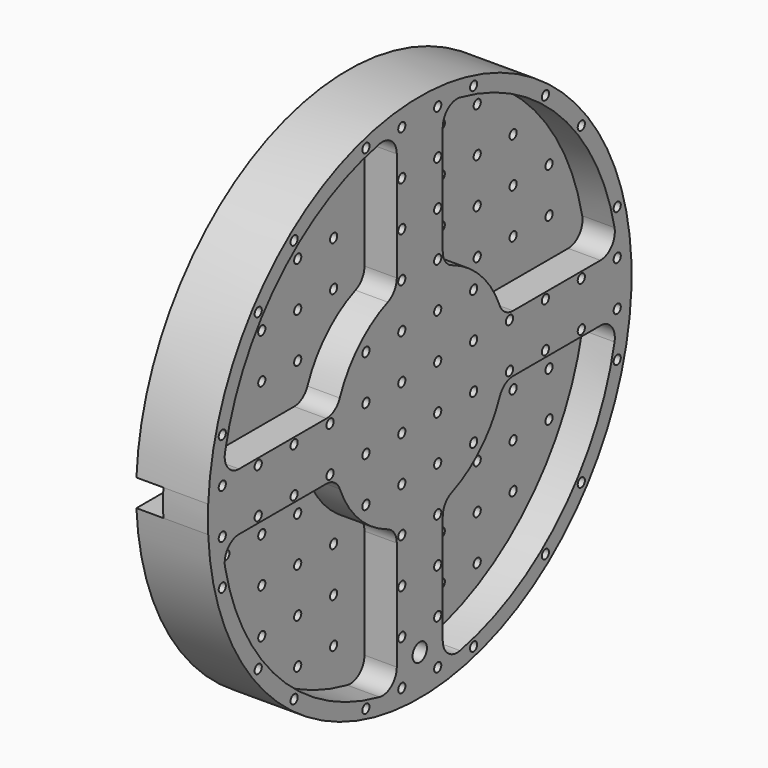
from build123d import *

# Parameters (mm, degrees)
F0_R     = 2.5
F0_R_2   = 5
F1_DEPTH = 40
F3_DEPTH = 15
F2_R     = 2.5
F4_DEPTH = 18


# Not quite as in the source:
# - a feature names something its author has since deleted; it is built from what else it names


with BuildPart() as f1:
    # F0 (on Right) → F1 (new body)
    with BuildSketch(Plane.YZ):
        with BuildLine():
            ThreePointArc((-147.3091986266, -7.5), (0, -147.5), (147.3091986266, -7.5))
            Line((147.3091986266, -7.5), (-147.3091986266, -7.5))
        make_face()
        with Locations((-87.5, -112.5)):
            Circle(F0_R, mode=Mode.SUBTRACT)
        with Locations((-112.5, -87.5)):
            Circle(F0_R, mode=Mode.SUBTRACT)
        with Locations((-87.5, -87.5)):
            Circle(F0_R, mode=Mode.SUBTRACT)
        with Locations((-37.5, -137.5)):
            Circle(F0_R, mode=Mode.SUBTRACT)
        with Locations((-62.5, -112.5)):
            Circle(F0_R, mode=Mode.SUBTRACT)
        with Locations((-37.5, -112.5)):
            Circle(F0_R, mode=Mode.SUBTRACT)
        with Locations((-12.5, -137.5)):
            Circle(F0_R, mode=Mode.SUBTRACT)
        with Locations((-12.5, -112.5)):
            Circle(F0_R, mode=Mode.SUBTRACT)
        with Locations((-62.5, -87.5)):
            Circle(F0_R, mode=Mode.SUBTRACT)
        with Locations((-37.5, -87.5)):
            Circle(F0_R, mode=Mode.SUBTRACT)
        with Locations((-12.5, -87.5)):
            Circle(F0_R, mode=Mode.SUBTRACT)
        with Locations((-112.5, -62.5)):
            Circle(F0_R, mode=Mode.SUBTRACT)
        with Locations((-137.5, -37.5)):
            Circle(F0_R, mode=Mode.SUBTRACT)
        with Locations((-112.5, -37.5)):
            Circle(F0_R, mode=Mode.SUBTRACT)
        with Locations((-87.5, -62.5)):
            Circle(F0_R, mode=Mode.SUBTRACT)
        with Locations((-87.5, -37.5)):
            Circle(F0_R, mode=Mode.SUBTRACT)
        with Locations((-137.5, -12.5)):
            Circle(F0_R, mode=Mode.SUBTRACT)
        with Locations((-112.5, -12.5)):
            Circle(F0_R, mode=Mode.SUBTRACT)
        with Locations((-87.5, -12.5)):
            Circle(F0_R, mode=Mode.SUBTRACT)
        with Locations((-62.5, -62.5)):
            Circle(F0_R, mode=Mode.SUBTRACT)
        with Locations((-37.5, -62.5)):
            Circle(F0_R, mode=Mode.SUBTRACT)
        with Locations((-62.5, -37.5)):
            Circle(F0_R, mode=Mode.SUBTRACT)
        with Locations((-37.5, -37.5)):
            Circle(F0_R, mode=Mode.SUBTRACT)
        with Locations((-12.5, -62.5)):
            Circle(F0_R, mode=Mode.SUBTRACT)
        with Locations((-12.5, -37.5)):
            Circle(F0_R, mode=Mode.SUBTRACT)
        with Locations((-62.5, -12.5)):
            Circle(F0_R, mode=Mode.SUBTRACT)
        with Locations((-37.5, -12.5)):
            Circle(F0_R, mode=Mode.SUBTRACT)
        with Locations((-12.5, -12.5)):
            Circle(F0_R, mode=Mode.SUBTRACT)
        with Locations((12.5, -137.5)):
            Circle(F0_R, mode=Mode.SUBTRACT)
        with Locations((0, -125)):
            Circle(F0_R_2, mode=Mode.SUBTRACT)
        with Locations((12.5, -112.5)):
            Circle(F0_R, mode=Mode.SUBTRACT)
        with Locations((37.5, -137.5)):
            Circle(F0_R, mode=Mode.SUBTRACT)
        with Locations((37.5, -112.5)):
            Circle(F0_R, mode=Mode.SUBTRACT)
        with Locations((62.5, -112.5)):
            Circle(F0_R, mode=Mode.SUBTRACT)
        with Locations((12.5, -87.5)):
            Circle(F0_R, mode=Mode.SUBTRACT)
        with Locations((37.5, -87.5)):
            Circle(F0_R, mode=Mode.SUBTRACT)
        with Locations((62.5, -87.5)):
            Circle(F0_R, mode=Mode.SUBTRACT)
        with Locations((87.5, -112.5)):
            Circle(F0_R, mode=Mode.SUBTRACT)
        with Locations((87.5, -87.5)):
            Circle(F0_R, mode=Mode.SUBTRACT)
        with Locations((112.5, -87.5)):
            Circle(F0_R, mode=Mode.SUBTRACT)
        with Locations((12.5, -62.5)):
            Circle(F0_R, mode=Mode.SUBTRACT)
        with Locations((12.5, -37.5)):
            Circle(F0_R, mode=Mode.SUBTRACT)
        with Locations((37.5, -62.5)):
            Circle(F0_R, mode=Mode.SUBTRACT)
        with Locations((62.5, -62.5)):
            Circle(F0_R, mode=Mode.SUBTRACT)
        with Locations((37.5, -37.5)):
            Circle(F0_R, mode=Mode.SUBTRACT)
        with Locations((62.5, -37.5)):
            Circle(F0_R, mode=Mode.SUBTRACT)
        with Locations((12.5, -12.5)):
            Circle(F0_R, mode=Mode.SUBTRACT)
        with Locations((37.5, -12.5)):
            Circle(F0_R, mode=Mode.SUBTRACT)
        with Locations((62.5, -12.5)):
            Circle(F0_R, mode=Mode.SUBTRACT)
        with Locations((87.5, -62.5)):
            Circle(F0_R, mode=Mode.SUBTRACT)
        with Locations((87.5, -37.5)):
            Circle(F0_R, mode=Mode.SUBTRACT)
        with Locations((112.5, -62.5)):
            Circle(F0_R, mode=Mode.SUBTRACT)
        with Locations((112.5, -37.5)):
            Circle(F0_R, mode=Mode.SUBTRACT)
        with Locations((137.5, -37.5)):
            Circle(F0_R, mode=Mode.SUBTRACT)
        with Locations((87.5, -12.5)):
            Circle(F0_R, mode=Mode.SUBTRACT)
        with Locations((112.5, -12.5)):
            Circle(F0_R, mode=Mode.SUBTRACT)
        with Locations((137.5, -12.5)):
            Circle(F0_R, mode=Mode.SUBTRACT)
        with BuildLine():
            Line((-147.3091986266, 7.5), (147.3091986266, 7.5))
            ThreePointArc((147.3091986266, 7.5), (0, 147.5), (-147.3091986266, 7.5))
        make_face()
        with Locations((-137.5, 12.5)):
            Circle(F0_R, mode=Mode.SUBTRACT)
        with Locations((-112.5, 12.5)):
            Circle(F0_R, mode=Mode.SUBTRACT)
        with Locations((-87.5, 12.5)):
            Circle(F0_R, mode=Mode.SUBTRACT)
        with Locations((-137.5, 37.5)):
            Circle(F0_R, mode=Mode.SUBTRACT)
        with Locations((-112.5, 37.5)):
            Circle(F0_R, mode=Mode.SUBTRACT)
        with Locations((-112.5, 62.5)):
            Circle(F0_R, mode=Mode.SUBTRACT)
        with Locations((-87.5, 37.5)):
            Circle(F0_R, mode=Mode.SUBTRACT)
        with Locations((-87.5, 62.5)):
            Circle(F0_R, mode=Mode.SUBTRACT)
        with Locations((-62.5, 12.5)):
            Circle(F0_R, mode=Mode.SUBTRACT)
        with Locations((-37.5, 12.5)):
            Circle(F0_R, mode=Mode.SUBTRACT)
        with Locations((-12.5, 12.5)):
            Circle(F0_R, mode=Mode.SUBTRACT)
        with Locations((-62.5, 37.5)):
            Circle(F0_R, mode=Mode.SUBTRACT)
        with Locations((-37.5, 37.5)):
            Circle(F0_R, mode=Mode.SUBTRACT)
        with Locations((-62.5, 62.5)):
            Circle(F0_R, mode=Mode.SUBTRACT)
        with Locations((-37.5, 62.5)):
            Circle(F0_R, mode=Mode.SUBTRACT)
        with Locations((-12.5, 37.5)):
            Circle(F0_R, mode=Mode.SUBTRACT)
        with Locations((-12.5, 62.5)):
            Circle(F0_R, mode=Mode.SUBTRACT)
        with Locations((-112.5, 87.5)):
            Circle(F0_R, mode=Mode.SUBTRACT)
        with Locations((-87.5, 87.5)):
            Circle(F0_R, mode=Mode.SUBTRACT)
        with Locations((-87.5, 112.5)):
            Circle(F0_R, mode=Mode.SUBTRACT)
        with Locations((-62.5, 87.5)):
            Circle(F0_R, mode=Mode.SUBTRACT)
        with Locations((-37.5, 87.5)):
            Circle(F0_R, mode=Mode.SUBTRACT)
        with Locations((-12.5, 87.5)):
            Circle(F0_R, mode=Mode.SUBTRACT)
        with Locations((-62.5, 112.5)):
            Circle(F0_R, mode=Mode.SUBTRACT)
        with Locations((-37.5, 112.5)):
            Circle(F0_R, mode=Mode.SUBTRACT)
        with Locations((-37.5, 137.5)):
            Circle(F0_R, mode=Mode.SUBTRACT)
        with Locations((-12.5, 112.5)):
            Circle(F0_R, mode=Mode.SUBTRACT)
        with Locations((-12.5, 137.5)):
            Circle(F0_R, mode=Mode.SUBTRACT)
        with Locations((12.5, 12.5)):
            Circle(F0_R, mode=Mode.SUBTRACT)
        with Locations((37.5, 12.5)):
            Circle(F0_R, mode=Mode.SUBTRACT)
        with Locations((62.5, 12.5)):
            Circle(F0_R, mode=Mode.SUBTRACT)
        with Locations((12.5, 37.5)):
            Circle(F0_R, mode=Mode.SUBTRACT)
        with Locations((12.5, 62.5)):
            Circle(F0_R, mode=Mode.SUBTRACT)
        with Locations((37.5, 37.5)):
            Circle(F0_R, mode=Mode.SUBTRACT)
        with Locations((62.5, 37.5)):
            Circle(F0_R, mode=Mode.SUBTRACT)
        with Locations((37.5, 62.5)):
            Circle(F0_R, mode=Mode.SUBTRACT)
        with Locations((62.5, 62.5)):
            Circle(F0_R, mode=Mode.SUBTRACT)
        with Locations((87.5, 12.5)):
            Circle(F0_R, mode=Mode.SUBTRACT)
        with Locations((112.5, 12.5)):
            Circle(F0_R, mode=Mode.SUBTRACT)
        with Locations((137.5, 12.5)):
            Circle(F0_R, mode=Mode.SUBTRACT)
        with Locations((87.5, 37.5)):
            Circle(F0_R, mode=Mode.SUBTRACT)
        with Locations((87.5, 62.5)):
            Circle(F0_R, mode=Mode.SUBTRACT)
        with Locations((112.5, 37.5)):
            Circle(F0_R, mode=Mode.SUBTRACT)
        with Locations((137.5, 37.5)):
            Circle(F0_R, mode=Mode.SUBTRACT)
        with Locations((112.5, 62.5)):
            Circle(F0_R, mode=Mode.SUBTRACT)
        with Locations((12.5, 87.5)):
            Circle(F0_R, mode=Mode.SUBTRACT)
        with Locations((37.5, 87.5)):
            Circle(F0_R, mode=Mode.SUBTRACT)
        with Locations((62.5, 87.5)):
            Circle(F0_R, mode=Mode.SUBTRACT)
        with Locations((12.5, 112.5)):
            Circle(F0_R, mode=Mode.SUBTRACT)
        with Locations((12.5, 137.5)):
            Circle(F0_R, mode=Mode.SUBTRACT)
        with Locations((37.5, 112.5)):
            Circle(F0_R, mode=Mode.SUBTRACT)
        with Locations((62.5, 112.5)):
            Circle(F0_R, mode=Mode.SUBTRACT)
        with Locations((37.5, 137.5)):
            Circle(F0_R, mode=Mode.SUBTRACT)
        with Locations((87.5, 87.5)):
            Circle(F0_R, mode=Mode.SUBTRACT)
        with Locations((112.5, 87.5)):
            Circle(F0_R, mode=Mode.SUBTRACT)
        with Locations((87.5, 112.5)):
            Circle(F0_R, mode=Mode.SUBTRACT)
        with BuildLine():
            ThreePointArc((147.3091986266, -7.5), (147.4522919412, -3.7512133092), (147.5, 0))
            ThreePointArc((147.5, 0), (147.4522919412, 3.7512133092), (147.3091986266, 7.5))
            Line((147.3091986266, 7.5), (-147.3091986266, 7.5))
            ThreePointArc((-147.3091986266, 7.5), (-147.5, 0), (-147.3091986266, -7.5))
            Line((-147.3091986266, -7.5), (147.3091986266, -7.5))
        make_face()
    extrude(amount=F1_DEPTH)

    # F0 (on Right) → F3 (cut)
    with BuildSketch(Plane.YZ):
        with BuildLine():
            ThreePointArc((147.3091986266, -7.5), (147.4522919412, -3.7512133092), (147.5, 0))
            ThreePointArc((147.5, 0), (147.4522919412, 3.7512133092), (147.3091986266, 7.5))
            Line((147.3091986266, 7.5), (-147.3091986266, 7.5))
            ThreePointArc((-147.3091986266, 7.5), (-147.5, 0), (-147.3091986266, -7.5))
            Line((-147.3091986266, -7.5), (147.3091986266, -7.5))
        make_face()
    extrude(amount=F3_DEPTH, mode=Mode.SUBTRACT)

    # F2 (on face) → F4 (cut)
    with BuildSketch(Plane.YZ.offset(40)):
        with BuildLine():
            ThreePointArc((-55.7076919175, 22.2857142857), (-42.4264068712, 42.4264068712), (-22.2857142857, 55.7076919175))
            ThreePointArc((-22.2857142857, 55.7076919175), (-17.7192132879, 59.3861881313), (-16, 64.9923072371))
            Line((-16, 64.9923072371), (-16, 125.8421630456))
            ThreePointArc((-16, 125.8421630456), (-19.6846798591, 133.5956610638), (-28.0233463035, 135.635327485))
            ThreePointArc((-28.0233463035, 135.635327485), (-97.9342891943, 97.9342891943), (-135.635327485, 28.0233463035))
            ThreePointArc((-135.635327485, 28.0233463035), (-135.6763281994, 27.8136139963), (-135.7128377786, 27.6030534351))
            ThreePointArc((-135.7128377786, 27.6030534351), (-133.4589384247, 19.5204372968), (-125.8421630456, 16))
            Line((-125.8421630456, 16), (-64.9923072371, 16))
            ThreePointArc((-64.9923072371, 16), (-59.3861881313, 17.7192132879), (-55.7076919175, 22.2857142857))
        make_face()
        with Locations((-112.5, 37.5)):
            Circle(F2_R, mode=Mode.SUBTRACT)
        with Locations((-112.5, 62.5)):
            Circle(F2_R, mode=Mode.SUBTRACT)
        with Locations((-87.5, 37.5)):
            Circle(F2_R, mode=Mode.SUBTRACT)
        with Locations((-87.5, 62.5)):
            Circle(F2_R, mode=Mode.SUBTRACT)
        with Locations((-62.5, 37.5)):
            Circle(F2_R, mode=Mode.SUBTRACT)
        with Locations((-62.5, 62.5)):
            Circle(F2_R, mode=Mode.SUBTRACT)
        with Locations((-37.5, 62.5)):
            Circle(F2_R, mode=Mode.SUBTRACT)
        with Locations((-87.5, 87.5)):
            Circle(F2_R, mode=Mode.SUBTRACT)
        with Locations((-62.5, 87.5)):
            Circle(F2_R, mode=Mode.SUBTRACT)
        with Locations((-37.5, 87.5)):
            Circle(F2_R, mode=Mode.SUBTRACT)
        with Locations((-62.5, 112.5)):
            Circle(F2_R, mode=Mode.SUBTRACT)
        with Locations((-37.5, 112.5)):
            Circle(F2_R, mode=Mode.SUBTRACT)
        with BuildLine():
            ThreePointArc((-125.8421630456, -16), (-133.5956610638, -19.6846798591), (-135.635327485, -28.0233463035))
            ThreePointArc((-135.635327485, -28.0233463035), (-97.9342891943, -97.9342891943), (-28.0233463035, -135.635327485))
            ThreePointArc((-28.0233463035, -135.635327485), (-19.6846798591, -133.5956610638), (-16, -125.8421630456))
            Line((-16, -125.8421630456), (-16, -64.9923072371))
            ThreePointArc((-16, -64.9923072371), (-17.7192132879, -59.3861881313), (-22.2857142857, -55.7076919175))
            ThreePointArc((-22.2857142857, -55.7076919175), (-42.4264068712, -42.4264068712), (-55.7076919175, -22.2857142857))
            ThreePointArc((-55.7076919175, -22.2857142857), (-59.3861881313, -17.7192132879), (-64.9923072371, -16))
            Line((-64.9923072371, -16), (-125.8421630456, -16))
        make_face()
        with Locations((-87.5, -87.5)):
            Circle(F2_R, mode=Mode.SUBTRACT)
        with Locations((-62.5, -112.5)):
            Circle(F2_R, mode=Mode.SUBTRACT)
        with Locations((-37.5, -112.5)):
            Circle(F2_R, mode=Mode.SUBTRACT)
        with Locations((-62.5, -87.5)):
            Circle(F2_R, mode=Mode.SUBTRACT)
        with Locations((-37.5, -87.5)):
            Circle(F2_R, mode=Mode.SUBTRACT)
        with Locations((-112.5, -62.5)):
            Circle(F2_R, mode=Mode.SUBTRACT)
        with Locations((-112.5, -37.5)):
            Circle(F2_R, mode=Mode.SUBTRACT)
        with Locations((-87.5, -62.5)):
            Circle(F2_R, mode=Mode.SUBTRACT)
        with Locations((-87.5, -37.5)):
            Circle(F2_R, mode=Mode.SUBTRACT)
        with Locations((-62.5, -62.5)):
            Circle(F2_R, mode=Mode.SUBTRACT)
        with Locations((-37.5, -62.5)):
            Circle(F2_R, mode=Mode.SUBTRACT)
        with Locations((-62.5, -37.5)):
            Circle(F2_R, mode=Mode.SUBTRACT)
        with BuildLine():
            ThreePointArc((22.2857142857, -55.7076919175), (17.7192132879, -59.3861881313), (16, -64.9923072371))
            Line((16, -64.9923072371), (16, -125.8421630456))
            ThreePointArc((16, -125.8421630456), (19.6846798591, -133.5956610638), (28.0233463035, -135.635327485))
            ThreePointArc((28.0233463035, -135.635327485), (97.9342891943, -97.9342891943), (135.635327485, -28.0233463035))
            ThreePointArc((135.635327485, -28.0233463035), (133.5956610638, -19.6846798591), (125.8421630456, -16))
            Line((125.8421630456, -16), (64.9923072371, -16))
            ThreePointArc((64.9923072371, -16), (59.3861881313, -17.7192132879), (55.7076919175, -22.2857142857))
            ThreePointArc((55.7076919175, -22.2857142857), (42.4264068712, -42.4264068712), (22.2857142857, -55.7076919175))
        make_face()
        with Locations((37.5, -112.5)):
            Circle(F2_R, mode=Mode.SUBTRACT)
        with Locations((62.5, -112.5)):
            Circle(F2_R, mode=Mode.SUBTRACT)
        with Locations((37.5, -87.5)):
            Circle(F2_R, mode=Mode.SUBTRACT)
        with Locations((62.5, -87.5)):
            Circle(F2_R, mode=Mode.SUBTRACT)
        with Locations((87.5, -87.5)):
            Circle(F2_R, mode=Mode.SUBTRACT)
        with Locations((37.5, -62.5)):
            Circle(F2_R, mode=Mode.SUBTRACT)
        with Locations((62.5, -62.5)):
            Circle(F2_R, mode=Mode.SUBTRACT)
        with Locations((62.5, -37.5)):
            Circle(F2_R, mode=Mode.SUBTRACT)
        with Locations((87.5, -62.5)):
            Circle(F2_R, mode=Mode.SUBTRACT)
        with Locations((87.5, -37.5)):
            Circle(F2_R, mode=Mode.SUBTRACT)
        with Locations((112.5, -62.5)):
            Circle(F2_R, mode=Mode.SUBTRACT)
        with Locations((112.5, -37.5)):
            Circle(F2_R, mode=Mode.SUBTRACT)
        with BuildLine():
            ThreePointArc((28.0233463035, 135.635327485), (19.6846798591, 133.5956610638), (16, 125.8421630456))
            Line((16, 125.8421630456), (16, 64.9923072371))
            ThreePointArc((16, 64.9923072371), (17.7192132879, 59.3861881313), (22.2857142857, 55.7076919175))
            ThreePointArc((22.2857142857, 55.7076919175), (42.4264068712, 42.4264068712), (55.7076919175, 22.2857142857))
            ThreePointArc((55.7076919175, 22.2857142857), (59.3861881313, 17.7192132879), (64.9923072371, 16))
            Line((64.9923072371, 16), (125.8421630456, 16))
            ThreePointArc((125.8421630456, 16), (133.5956610638, 19.6846798591), (135.635327485, 28.0233463035))
            ThreePointArc((135.635327485, 28.0233463035), (97.9342891943, 97.9342891943), (28.0233463035, 135.635327485))
        make_face()
        with Locations((62.5, 37.5)):
            Circle(F2_R, mode=Mode.SUBTRACT)
        with Locations((37.5, 62.5)):
            Circle(F2_R, mode=Mode.SUBTRACT)
        with Locations((62.5, 62.5)):
            Circle(F2_R, mode=Mode.SUBTRACT)
        with Locations((87.5, 37.5)):
            Circle(F2_R, mode=Mode.SUBTRACT)
        with Locations((87.5, 62.5)):
            Circle(F2_R, mode=Mode.SUBTRACT)
        with Locations((112.5, 37.5)):
            Circle(F2_R, mode=Mode.SUBTRACT)
        with Locations((112.5, 62.5)):
            Circle(F2_R, mode=Mode.SUBTRACT)
        with Locations((37.5, 87.5)):
            Circle(F2_R, mode=Mode.SUBTRACT)
        with Locations((62.5, 87.5)):
            Circle(F2_R, mode=Mode.SUBTRACT)
        with Locations((37.5, 112.5)):
            Circle(F2_R, mode=Mode.SUBTRACT)
        with Locations((62.5, 112.5)):
            Circle(F2_R, mode=Mode.SUBTRACT)
        with Locations((87.5, 87.5)):
            Circle(F2_R, mode=Mode.SUBTRACT)
    extrude(amount=-F4_DEPTH, mode=Mode.SUBTRACT)


solid = f1.part
